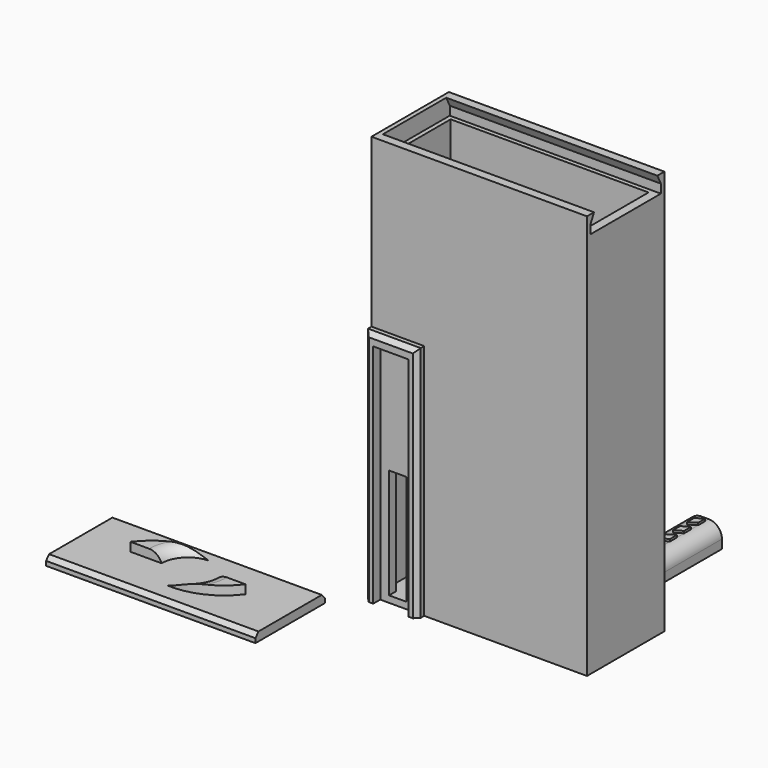
from build123d import *

# Parameters (mm, degrees)
F0_W         = 49
F0_H         = 22
F0_W_2       = 45
F0_H_2       = 18
F1_DEPTH     = 88
F2_DEPTH     = 3
F3_W         = 4
F3_H         = 25
F4_DEPTH     = 20
F5_DEPTH     = 1.5
F6_W         = 2
F6_H         = 50
F6_H_2       = 1.5
F7_DEPTH     = 2
F8_T1_DEPTH  = 17.1433659759
F8_T3_DEPTH  = 59.1433659759
F10_DEPTH    = 1.5
F9_W         = 3.7
F9_H         = 6
F9_H_2       = 1.5
F11_DEPTH    = 2
F9_W_2       = 7.7
F9_H_3       = 27.5
F12_DEPTH    = 5
F13_DEPTH    = 2.5
F14_R        = 3
F16_DEPTH    = 0.5
F18_DEPTH    = 32.1
F19_DEPTH    = 4
F21_DEPTH    = 48
F22_W        = 47.6
F22_H        = 19.7
F23_DEPTH    = 2
F25_DEPTH    = 49
F27_DEPTH    = 2
F28_T2_ANGLE = 271.3601385913
F28_T4_ANGLE = 271.3601385913


# Not quite as in the source:
# - a fillet or chamfer that OpenCascade refuses, or shapes differently, is made with other operations: its cross-section is extruded or revolved along the edge and cut away or added


with BuildPart() as f1:
    # F0 (on Top) → F1 (new body)
    with BuildSketch(Plane.XY):
        Rectangle(F0_W, F0_H)
        Rectangle(F0_W_2, F0_H_2, mode=Mode.SUBTRACT)
    extrude(amount=F1_DEPTH)

    # F0 (on Top) → F2 (join)
    with BuildSketch(Plane.XY):
        Rectangle(F0_W_2, F0_H_2)
    extrude(amount=F2_DEPTH)

    # F3 (on face) → F4 (cut)
    with BuildSketch(Plane.XZ.offset(11)):
        with Locations((-18.5, 14)):
            Rectangle(F3_W, F3_H)
    extrude(amount=-F4_DEPTH, mode=Mode.SUBTRACT)

    # F5 (cut): a face of the model
    f5_faces = [f1.faces().sort_by_distance(p)[0] for p in [
        (-21.5, 0, 3),
    ]]
    extrude(f5_faces, amount=-F5_DEPTH, mode=Mode.SUBTRACT)

    # F6 (on face) → F7 (join)
    with BuildSketch(Plane.XZ.offset(11)):
        with Locations((-23.5, 26.5)):
            Rectangle(F6_W, F6_H)
        Polygon((-24.5, 51.5), (-22.5, 51.5), (-14.5, 51.5), (-12.5, 51.5), (-12.5, 54), (-24.5, 54), align=None)
        with Locations((-13.5, 26.5)):
            Rectangle(F6_W, F6_H)
        with Locations((-23.5, 0.75)):
            Rectangle(F6_W, F6_H_2)
        with Locations((-13.5, 0.75)):
            Rectangle(F6_W, F6_H_2)
    extrude(amount=F7_DEPTH)

    # F8: chamfer of 1 on 5 edges, made by hand

    # F8_s2 → F8_t1 (cut)
    with BuildSketch(Plane.YZ.offset(-27.071682988)):
        Polygon((-13, 53), (-12, 54), (-13, 54), align=None)
    extrude(amount=F8_T1_DEPTH, mode=Mode.SUBTRACT)

    # F8_s4 → F8_t3 (cut)
    with BuildSketch(Plane.XY.offset(-2.571682988)):
        Polygon((-23.5, -13), (-24.5, -12), (-24.5, -13), align=None)
        Polygon((-13.5, -13), (-12.5, -12), (-12.5, -13), align=None)
    extrude(amount=F8_T3_DEPTH, mode=Mode.SUBTRACT)

    # F17 (on face) → F19 (join)
    with BuildSketch(Plane.XY.offset(88)):
        Polygon((-23.5, 10), (-22.5, 10), (22.5, 10), (24.5, 10), (24.5, 11), (-24.5, 11), (-24.5, -11), (24.5, -11), (24.5, -10), (22.5, -10), (-22.5, -10), (-23.5, -10), align=None)
    extrude(amount=F19_DEPTH)

    # F20 (on face) → F21 (join)
    with BuildSketch(Plane.YZ.offset(-23.5)):
        Polygon((-9, 92), (-10, 92), (-10, 90), align=None)
        Polygon((10, 92), (9, 92), (10, 90), align=None)
    extrude(amount=F21_DEPTH)


with BuildPart() as f10:
    # F9 (on Top) → F10 (new body)
    with BuildSketch(Plane.XY):
        Polygon((-15.8205656037, 22.0463685691), (-15.8205656037, 39.0463685691), (-21.3205656037, 39.0463685691), (-21.3205656037, 22.0463685691), (-19.5205656037, 22.0463685691), align=None)
    extrude(amount=F10_DEPTH)

    # F9 (on Top) → F11 (join)
    with BuildSketch(Plane.XY):
        with Locations((-17.6705656037, 17.5463685691)):
            Rectangle(F9_W, F9_H)
        with Locations((-17.6705656037, 21.2963685691)):
            Rectangle(F9_W, F9_H_2)
    extrude(amount=F11_DEPTH)


with BuildPart() as f12:
    # F9 (on Top) → F12 (new body)
    with BuildSketch(Plane.XY):
        with Locations((8.8597331405, 28.3340272307)):
            Rectangle(F9_W_2, F9_H_3)
        Polygon((11.1597331405, 16.0840272307), (8.8597331405, 16.0840272307), (6.5597331405, 16.0840272307), (6.5597331405, 18.0840272307), (11.1597331405, 18.0840272307), align=None, mode=Mode.SUBTRACT)
        Polygon((6.5597331405, 16.0840272307), (8.8597331405, 16.0840272307), (11.1597331405, 16.0840272307), (11.1597331405, 18.0840272307), (6.5597331405, 18.0840272307), align=None)
    extrude(amount=F12_DEPTH)

    # F9 (on Top) → F13 (cut)
    with BuildSketch(Plane.XY):
        Polygon((6.5597331405, 16.0840272307), (8.8597331405, 16.0840272307), (11.1597331405, 16.0840272307), (11.1597331405, 18.0840272307), (6.5597331405, 18.0840272307), align=None)
    extrude(amount=F13_DEPTH, mode=Mode.SUBTRACT)

    # F14
    f14_edges = [f12.edges().sort_by_distance(p)[0] for p in [
        (5.009733, 28.334027, 5),
        (12.709733, 28.334027, 5),
    ]]
    fillet(f14_edges, radius=F14_R)

    # F15 (on face) → F16 (join)
    with BuildSketch(Plane.XY.offset(5)):
        Polygon((9.7097331405, 39.0840272307), (9.7097331405, 41.0840272307), (8.0097331405, 40.0840272307), align=None)
        Polygon((9.7097331405, 39.0840272307), (8.0097331405, 40.0840272307), (8.0097331405, 39.0840272307), (8.0097331405, 38.0840272307), align=None)
        Polygon((9.7097331405, 35.0840272307), (9.7097331405, 37.0840272307), (8.0097331405, 36.0840272307), align=None)
        Polygon((9.7097331405, 35.0840272307), (8.0097331405, 36.0840272307), (8.0097331405, 35.0840272307), (8.0097331405, 34.0840272307), align=None)
        Polygon((9.7097331405, 31.0840272307), (9.7097331405, 33.0840272307), (8.0097331405, 32.0840272307), align=None)
        Polygon((9.7097331405, 31.0840272307), (8.0097331405, 32.0840272307), (8.0097331405, 31.0840272307), (8.0097331405, 30.0840272307), align=None)
        Polygon((9.7097331405, 27.0840272307), (9.7097331405, 29.0840272307), (8.0097331405, 28.0840272307), align=None)
        Polygon((9.7097331405, 27.0840272307), (8.0097331405, 28.0840272307), (8.0097331405, 27.0840272307), (8.0097331405, 26.0840272307), align=None)
        Polygon((9.7097331405, 23.0840272307), (9.7097331405, 25.0840272307), (8.0097331405, 24.0840272307), align=None)
        Polygon((9.7097331405, 23.0840272307), (8.0097331405, 24.0840272307), (8.0097331405, 23.0840272307), (8.0097331405, 22.0840272307), align=None)
        Polygon((9.7097331405, 19.0840272307), (9.7097331405, 21.0840272307), (8.0097331405, 20.0840272307), align=None)
        Polygon((9.7097331405, 19.0840272307), (8.0097331405, 20.0840272307), (8.0097331405, 19.0840272307), (8.0097331405, 18.0840272307), align=None)
        Polygon((9.7097331405, 15.0840272307), (9.7097331405, 17.0840272307), (8.0097331405, 16.0840272307), align=None)
        Polygon((9.7097331405, 15.0840272307), (8.0097331405, 16.0840272307), (8.0097331405, 15.0840272307), align=None)
    extrude(amount=F16_DEPTH)

    # F9 (on Top) → F18 (cut)
    with BuildSketch(Plane.XY):
        Polygon((6.5597331405, 16.0840272307), (8.8597331405, 16.0840272307), (11.1597331405, 16.0840272307), (11.1597331405, 18.0840272307), (6.5597331405, 18.0840272307), align=None)
    extrude(amount=F18_DEPTH, mode=Mode.SUBTRACT)


with BuildPart() as f23:
    # F22 (on Top) → F23 (new body)
    with BuildSketch(Plane.XY):
        with Locations((-53.1354887307, -28.0733844578)):
            Rectangle(F22_W, F22_H)
    extrude(amount=F23_DEPTH)

    # F24 (on face) → F25 (cut)
    with BuildSketch(Plane.YZ.offset(-29.3354887307)):
        Polygon((-37.9233844578, 1), (-37.0733844578, 2), (-37.9233844578, 2), align=None)
        Polygon((-18.2233844578, 2), (-19.0733844578, 2), (-18.2233844578, 1), align=None)
    extrude(amount=-F25_DEPTH, mode=Mode.SUBTRACT)

    # F26 (on face) → F27 (join)
    with BuildSketch(Plane.XY.offset(2)):
        with BuildLine():
            ThreePointArc((-53.195998495, -21.3306639587), (-60.4566809918, -22.7037450747), (-66.2064477801, -27.34519355))
            Line((-66.2064477801, -27.34519355), (-59.1503226965, -27.34519355))
            ThreePointArc((-59.1503226965, -27.34519355), (-57.5267238276, -23.2348064685), (-53.532451262, -21.3434730979))
            ThreePointArc((-53.532451262, -21.3434730979), (-53.3643145243, -21.334713836), (-53.195998495, -21.3306639587))
        make_face()
        with BuildLine():
            ThreePointArc((-47.1206547649, -27.34519355), (-48.8610189494, -31.5768759253), (-53.0749789663, -33.3597231413))
            ThreePointArc((-53.0749789663, -33.3597231413), (-45.8142964696, -31.9866420253), (-40.0645296812, -27.34519355))
            Line((-40.0645296812, -27.34519355), (-47.1206547649, -27.34519355))
        make_face()
    extrude(amount=F27_DEPTH)

    # F28: fillet of radius 3 on 2 edges, made by hand

    # F28_s1 → F28_t2 (revolve, cut)
    with BuildSketch(Plane(origin=(-35.5706079716, 14.8183384522, 0), x_dir=(0, 0, 1), z_dir=(0.9231022415, -0.3845546146, 0))):
        with BuildLine():
            ThreePointArc((2, 51.6907408203), (3.4494897428, 52.7871171375), (4, 54.519167945))
            Line((4, 54.519167945), (4, 51.6907408203))
            Line((4, 51.6907408203), (2, 51.6907408203))
        make_face()
    revolve(axis=Axis((-53.1354887307, -27.34519355, 4), (0, 0, -1)), revolution_arc=F28_T2_ANGLE, mode=Mode.SUBTRACT)

    # F28_s3 → F28_t4 (revolve, cut)
    with BuildSketch(Plane(origin=(-35.5706079716, 14.8183384522, 0), x_dir=(0, 0, 1), z_dir=(-0.9231022415, 0.3845546146, 0))):
        with BuildLine():
            ThreePointArc((2, -39.6610728887), (3.4494897428, -38.5646965715), (4, -36.8326457639))
            Line((4, -36.8326457639), (4, -39.6610728887))
            Line((4, -39.6610728887), (2, -39.6610728887))
        make_face()
    revolve(axis=Axis((-53.1354887307, -27.34519355, 4), (0, 0, -1)), revolution_arc=F28_T4_ANGLE, mode=Mode.SUBTRACT)


solid = Compound([f1.part, f10.part, f12.part, f23.part])
